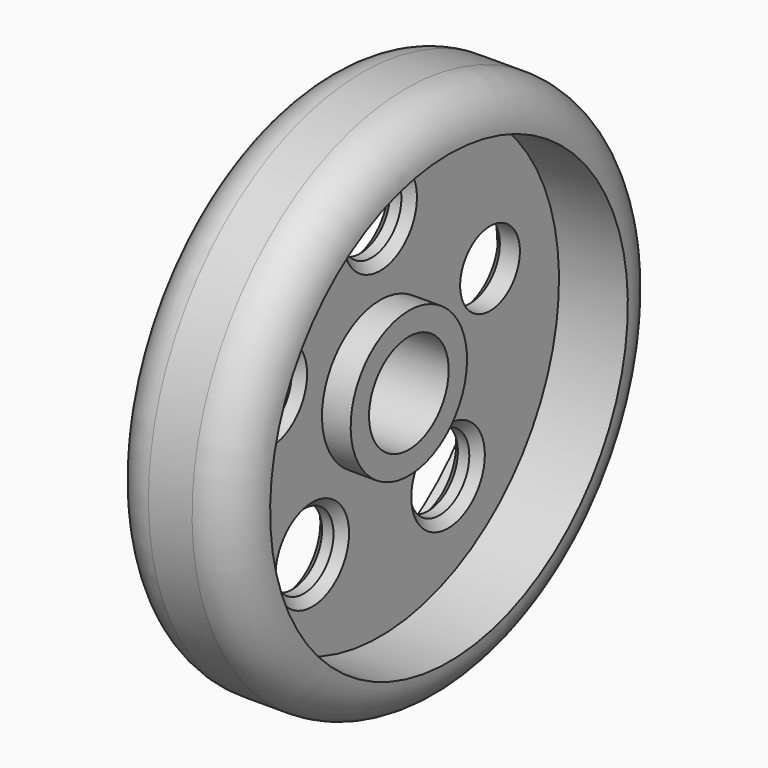
from build123d import *

# Parameters (mm, degrees)
F3_D     = 8.654
F3_DEPTH = 10
F3_TIP   = 2.5999238985
F4_R     = 5
F5_SIZE  = 1


with BuildPart() as f1:
    # F0 (on Front) → F1 (revolve)
    with BuildSketch(Plane.XZ):
        Polygon((15.0574529544, 30.9514049441), (0, 30.9514049441), (0, 25.9012449533), (3.761041211, 25.9012449533), (3.761041211, 8.42503272), (0, 8.42503272), (0, 5.7670525275), (10.4059893638, 5.7670525275), (10.4059893638, 8.42503272), (7.0835147053, 8.42503272), (7.0835147053, 25.9012449533), (15.0574529544, 25.9012449533), align=None)
    revolve(axis=Axis((5.2029946819, 0, 0), (1, 0, 0)))

    # F3
    with Locations(Plane(origin=(3.761041211, 0, 0), x_dir=(0, -1, 0), z_dir=(-1, 0, 0))):
        with Locations((-15.9109056188, 5.1697666204), (0, 16.7297162116), (15.9109056188, 5.1697666204), (9.8334804642, -13.5346247262), (-9.8334804642, -13.5346247262)):
            Hole(F3_D / 2, depth=F3_DEPTH)
            with Locations((0, 0, -(F3_DEPTH + F3_TIP / 2))):  # 118° drill point
                Cone(0, F3_D / 2, F3_TIP, mode=Mode.SUBTRACT)

    # F4
    f4_edges = [f1.edges().sort_by_distance(p)[0] for p in [
        (0, 0, -30.951405),
        (15.057453, 0, -30.951405),
    ]]
    fillet(f4_edges, radius=F4_R)

    # F5
    f5_edges = [f1.edges().sort_by_distance(p)[0] for p in [
        (0, 0, -8.425033),
        (0, 0, -5.767053),
        (7.083515, 4.327, 16.729716),
        (7.083515, 14.16048, -13.534625),
        (7.083515, -11.583906, 5.169767),
        (7.083515, -5.50648, -13.534625),
        (3.761041, 14.16048, -13.534625),
        (3.761041, 20.237906, 5.169767),
        (3.761041, 4.327, 16.729716),
        (3.761041, -5.50648, -13.534625),
        (3.761041, -11.583906, 5.169767),
    ]]
    chamfer(f5_edges, length=F5_SIZE)


solid = f1.part
